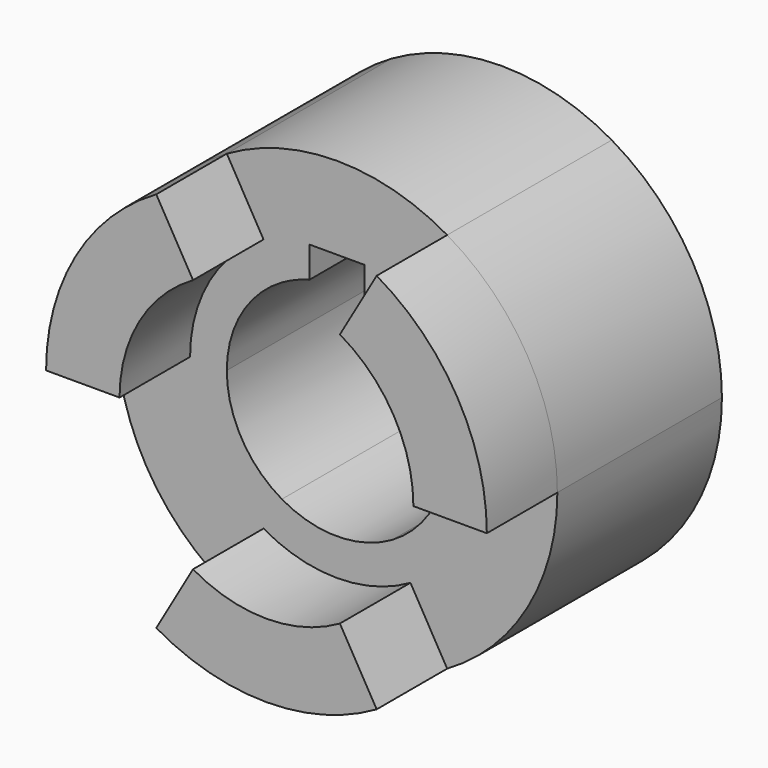
from build123d import *

# Parameters (mm, degrees)
F1_DEPTH = 8.89
F2_DEPTH = 3.81


with BuildPart() as f1:
    # F0 (on Front) → F1 (new body)
    with BuildSketch(Plane.XZ):
        with BuildLine():
            Line((6.35, 0), (9.525, 0))
            ThreePointArc((9.525, 0), (8.248891971, 4.7625), (4.7625, 8.248891971))
            Line((4.7625, 8.248891971), (3.175, 5.499261314))
            ThreePointArc((3.175, 5.499261314), (5.499261314, 3.175), (6.35, 0))
        make_face()
        with BuildLine():
            Line((3.175, 5.499261314), (4.7625, 8.248891971))
            ThreePointArc((4.7625, 8.248891971), (0, 9.525), (-4.7625, 8.248891971))
            Line((-4.7625, 8.248891971), (-3.175, 5.499261314))
            ThreePointArc((-3.175, 5.499261314), (0, 6.35), (3.175, 5.499261314))
        make_face()
        with BuildLine():
            Line((4.7625, 0), (6.35, 0))
            ThreePointArc((6.35, 0), (5.499261314, 3.175), (3.175, 5.499261314))
            Line((3.175, 5.499261314), (2.38125, 4.1244459855))
            ThreePointArc((2.38125, 4.1244459855), (4.1244459855, 2.38125), (4.7625, 0))
        make_face()
        with BuildLine():
            Line((2.38125, 4.1244459855), (3.175, 5.499261314))
            ThreePointArc((3.175, 5.499261314), (0, 6.35), (-3.175, 5.499261314))
            Line((-3.175, 5.499261314), (-2.38125, 4.1244459855))
            ThreePointArc((-2.38125, 4.1244459855), (-1.8024489876, 4.4082404536), (-1.190625, 4.6112707966))
            Line((-1.190625, 4.6112707966), (-1.190625, 5.953125))
            Line((-1.190625, 5.953125), (1.190625, 5.953125))
            Line((1.190625, 5.953125), (1.190625, 4.6112707966))
            ThreePointArc((1.190625, 4.6112707966), (1.8024489876, 4.4082404536), (2.38125, 4.1244459855))
        make_face()
        with BuildLine():
            ThreePointArc((4.7625, -8.248891971), (8.248891971, -4.7625), (9.525, 0))
            Line((9.525, 0), (6.35, 0))
            ThreePointArc((6.35, 0), (5.499261314, -3.175), (3.175, -5.499261314))
            Line((3.175, -5.499261314), (4.7625, -8.248891971))
        make_face()
        with BuildLine():
            Line((-2.38125, 4.1244459855), (-3.175, 5.499261314))
            ThreePointArc((-3.175, 5.499261314), (-5.499261314, 3.175), (-6.35, 0))
            Line((-6.35, 0), (-4.7625, 0))
            ThreePointArc((-4.7625, 0), (-4.1244459855, 2.38125), (-2.38125, 4.1244459855))
        make_face()
        with BuildLine():
            ThreePointArc((-6.35, 0), (-5.499261314, -3.175), (-3.175, -5.499261314))
            Line((-3.175, -5.499261314), (-2.38125, -4.1244459855))
            ThreePointArc((-2.38125, -4.1244459855), (-4.1244459855, -2.38125), (-4.7625, 0))
            Line((-4.7625, 0), (-6.35, 0))
        make_face()
        with BuildLine():
            ThreePointArc((-9.525, 0), (-8.248891971, -4.7625), (-4.7625, -8.248891971))
            Line((-4.7625, -8.248891971), (-3.175, -5.499261314))
            ThreePointArc((-3.175, -5.499261314), (-5.499261314, -3.175), (-6.35, 0))
            Line((-6.35, 0), (-9.525, 0))
        make_face()
        with BuildLine():
            ThreePointArc((-4.7625, -8.248891971), (0, -9.525), (4.7625, -8.248891971))
            Line((4.7625, -8.248891971), (3.175, -5.499261314))
            ThreePointArc((3.175, -5.499261314), (0, -6.35), (-3.175, -5.499261314))
            Line((-3.175, -5.499261314), (-4.7625, -8.248891971))
        make_face()
        with BuildLine():
            ThreePointArc((-3.175, -5.499261314), (0, -6.35), (3.175, -5.499261314))
            Line((3.175, -5.499261314), (2.38125, -4.1244459855))
            ThreePointArc((2.38125, -4.1244459855), (0, -4.7625), (-2.38125, -4.1244459855))
            Line((-2.38125, -4.1244459855), (-3.175, -5.499261314))
        make_face()
        with BuildLine():
            ThreePointArc((3.175, -5.499261314), (5.499261314, -3.175), (6.35, 0))
            Line((6.35, 0), (4.7625, 0))
            ThreePointArc((4.7625, 0), (4.1244459855, -2.38125), (2.38125, -4.1244459855))
            Line((2.38125, -4.1244459855), (3.175, -5.499261314))
        make_face()
        with BuildLine():
            Line((-3.175, 5.499261314), (-4.7625, 8.248891971))
            ThreePointArc((-4.7625, 8.248891971), (-8.248891971, 4.7625), (-9.525, 0))
            Line((-9.525, 0), (-6.35, 0))
            ThreePointArc((-6.35, 0), (-5.499261314, 3.175), (-3.175, 5.499261314))
        make_face()
    extrude(amount=-F1_DEPTH)

    # F0 (on Front) → F2 (join)
    with BuildSketch(Plane.XZ):
        with BuildLine():
            Line((6.35, 0), (9.525, 0))
            ThreePointArc((9.525, 0), (8.248891971, 4.7625), (4.7625, 8.248891971))
            Line((4.7625, 8.248891971), (3.175, 5.499261314))
            ThreePointArc((3.175, 5.499261314), (5.499261314, 3.175), (6.35, 0))
        make_face()
        with BuildLine():
            ThreePointArc((-4.7625, -8.248891971), (0, -9.525), (4.7625, -8.248891971))
            Line((4.7625, -8.248891971), (3.175, -5.499261314))
            ThreePointArc((3.175, -5.499261314), (0, -6.35), (-3.175, -5.499261314))
            Line((-3.175, -5.499261314), (-4.7625, -8.248891971))
        make_face()
        with BuildLine():
            Line((-3.175, 5.499261314), (-4.7625, 8.248891971))
            ThreePointArc((-4.7625, 8.248891971), (-8.248891971, 4.7625), (-9.525, 0))
            Line((-9.525, 0), (-6.35, 0))
            ThreePointArc((-6.35, 0), (-5.499261314, 3.175), (-3.175, 5.499261314))
        make_face()
    extrude(amount=F2_DEPTH)


solid = f1.part
